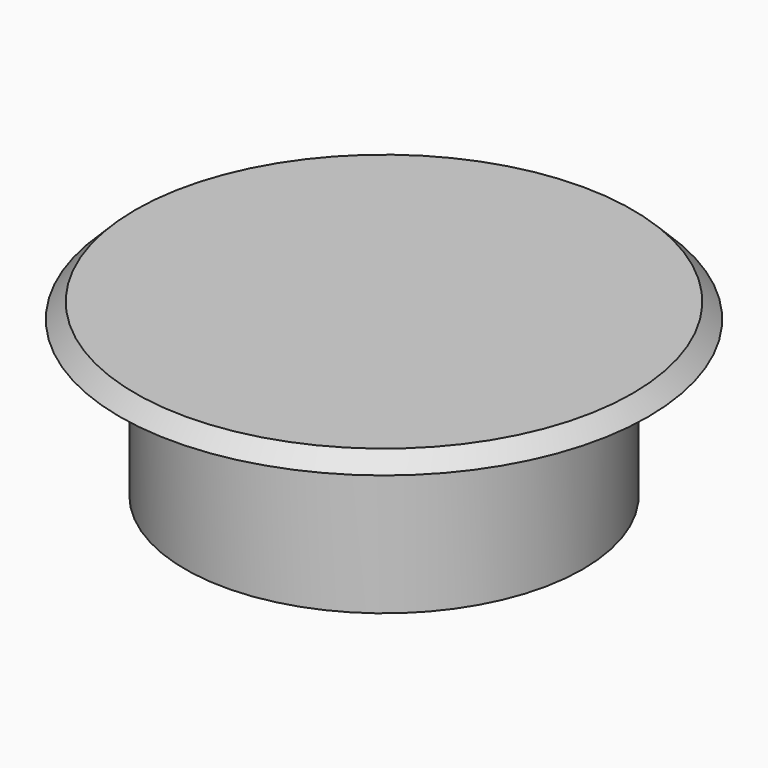
from build123d import *

# Parameters (mm, degrees)
F0_W     = 1.2
F0_H     = 10
F4_DEPTH = 10


# Not quite as in the source:
# - a fillet or chamfer that OpenCascade refuses, or shapes differently, is made with other operations: its cross-section is extruded or revolved along the edge and cut away or added


with BuildPart() as f1:
    # F0 (on Front) → F1 (revolve)
    with BuildSketch(Plane.XZ):
        Polygon((0, 11), (0, 10), (11.6, 10), (12.8, 10), (18, 10), (18, 11), align=None)
        with Locations((12.2, 5)):
            Rectangle(F0_W, F0_H)
    revolve(axis=Axis((0, 0, 10.5), (0, 0, -1)))

    # F2: chamfer of 2 on 1 edges, made by hand

    # F2_s1 → F2_t2 (revolve, cut)
    with BuildSketch(Plane.XZ):
        Polygon((18, 9), (16, 11), (18, 11), align=None)
    revolve(axis=Axis((0, 0, 11), (0, 0, -1)), mode=Mode.SUBTRACT)


with BuildPart() as f4:
    # F3 (on face) → F4 (new body)
    with BuildSketch(Plane(origin=(0, 0, 10), x_dir=(1, 0, 0), z_dir=(0, 0, -1))):
        Polygon((-11.4316838985, 1.9689091509), (-11.5669518457, 0.875), (11.5669518457, 0.875), (11.4316838985, 1.9689091509), align=None)
    extrude(amount=F4_DEPTH)


with BuildPart() as f4b:
    # F3 (on face) → F4, piece 2 (new body)
    with BuildSketch(Plane(origin=(0, 0, 10), x_dir=(1, 0, 0), z_dir=(0, 0, -1))):
        Polygon((11.5669518457, -0.875), (-11.5669518457, -0.875), (-11.421984153, -2.0244204128), (11.421984153, -2.0244204128), align=None)
    extrude(amount=F4_DEPTH)


solid = Compound([f1.part, f4.part, f4b.part])
